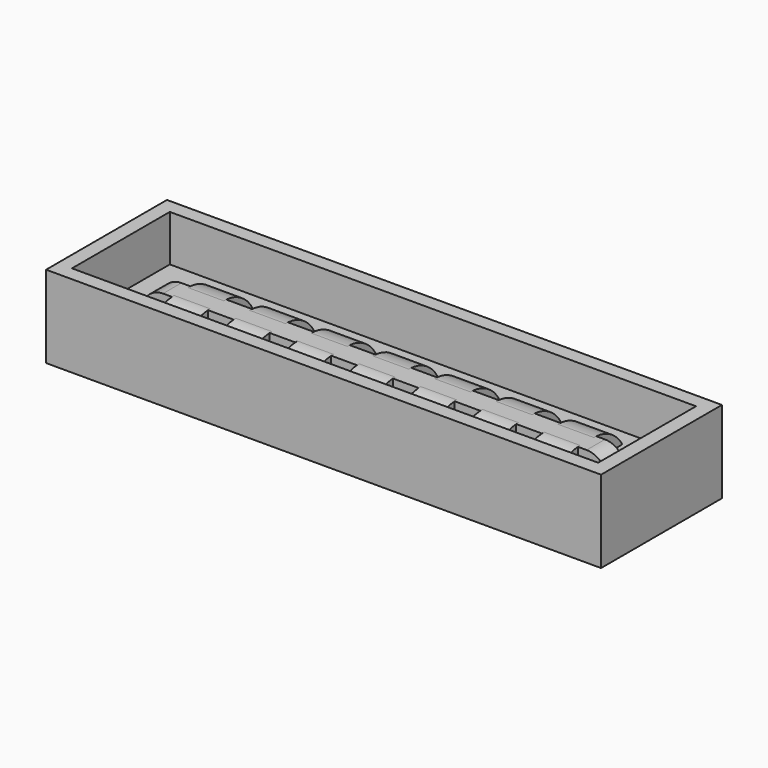
from build123d import *

# Parameters (mm, degrees)
F0_W         = 137.16
F0_H         = 37.338
F1_DEPTH     = 20.32
F2_W         = 130.048
F2_H         = 30.226
F3_DEPTH     = 11.43
F4_W         = 8.89
F4_H         = 21.844
F5_DEPTH     = 5.08
F6_T1_DEPTH  = 30.8870452561
F6_T3_DEPTH  = 52.8840905123
F6_T5_DEPTH  = 52.8840905123
F6_T7_DEPTH  = 52.8840905123
F6_T9_DEPTH  = 52.8840905123
F6_T11_DEPTH = 52.8840905123
F6_T13_DEPTH = 30.8870452561
F7_W         = 7.2538567698
F7_H         = 5.6681656279
F7_W_2       = 6.35
F8_DEPTH     = 5.08
F9_R         = 5.07999


# Not quite as in the source:
# - a fillet or chamfer that OpenCascade refuses, or shapes differently, is made with other operations: its cross-section is extruded or revolved along the edge and cut away or added
# - a fillet or chamfer is up to 0.001 mm smaller than in the source, because OpenCascade refuses the exact size
# - a feature names something its author has since deleted; it is built from what else it names


with BuildPart() as f1:
    # F0 (on Top) → F1 (new body)
    with BuildSketch(Plane.XY):
        Rectangle(F0_W, F0_H)
    extrude(amount=F1_DEPTH)

    # F2 (on face) → F3 (cut)
    with BuildSketch(Plane.XY.offset(20.32)):
        Rectangle(F2_W, F2_H)
    extrude(amount=-F3_DEPTH, mode=Mode.SUBTRACT)

    # F4 (on face) → F5 (join)
    with BuildSketch(Plane.XY.offset(8.89)):
        Rectangle(F4_W, F4_H)
        with Locations((15.24, 0)):
            Rectangle(F4_W, F4_H)
        with Locations((30.48, 0)):
            Rectangle(F4_W, F4_H)
        with Locations((45.72, 0)):
            Rectangle(F4_W, F4_H)
        with Locations((-15.24, 0)):
            Rectangle(F4_W, F4_H)
        with Locations((-30.48, 0)):
            Rectangle(F4_W, F4_H)
        with Locations((-45.72, 0)):
            Rectangle(F4_W, F4_H)
    extrude(amount=F5_DEPTH)

    # F6: fillet of radius 10.16 on 14 edges, made by hand

    # F6_s2 → F6_t1 (cut)
    with BuildSketch(Plane.YZ.offset(-50.165)):
        with BuildLine():
            ThreePointArc((-10.922, 8.89), (-7.2031818975, 12.6088181024), (-2.1231818975, 13.97))
            Line((-2.1231818975, 13.97), (-10.922, 13.97))
            Line((-10.922, 13.97), (-10.922, 8.89))
        make_face()
        with BuildLine():
            ThreePointArc((10.922, 8.89), (7.2031818975, 12.6088181024), (2.1231818975, 13.97))
            Line((2.1231818975, 13.97), (10.922, 13.97))
            Line((10.922, 13.97), (10.922, 8.89))
        make_face()
    extrude(amount=F6_T1_DEPTH, mode=Mode.SUBTRACT)

    # F6_s4 → F6_t3 (cut)
    with BuildSketch(Plane.YZ.offset(-56.9220452561)):
        with BuildLine():
            ThreePointArc((-10.922, 8.89), (-7.2031818975, 12.6088181024), (-2.1231818975, 13.97))
            Line((-2.1231818975, 13.97), (-10.922, 13.97))
            Line((-10.922, 13.97), (-10.922, 8.89))
        make_face()
        with BuildLine():
            ThreePointArc((10.922, 8.89), (7.2031818975, 12.6088181024), (2.1231818975, 13.97))
            Line((2.1231818975, 13.97), (10.922, 13.97))
            Line((10.922, 13.97), (10.922, 8.89))
        make_face()
    extrude(amount=F6_T3_DEPTH, mode=Mode.SUBTRACT)

    # F6_s6 → F6_t5 (cut)
    with BuildSketch(Plane.YZ.offset(-41.6820452561)):
        with BuildLine():
            ThreePointArc((-10.922, 8.89), (-7.2031818975, 12.6088181024), (-2.1231818975, 13.97))
            Line((-2.1231818975, 13.97), (-10.922, 13.97))
            Line((-10.922, 13.97), (-10.922, 8.89))
        make_face()
        with BuildLine():
            ThreePointArc((10.922, 8.89), (7.2031818975, 12.6088181024), (2.1231818975, 13.97))
            Line((2.1231818975, 13.97), (10.922, 13.97))
            Line((10.922, 13.97), (10.922, 8.89))
        make_face()
    extrude(amount=F6_T5_DEPTH, mode=Mode.SUBTRACT)

    # F6_s8 → F6_t7 (cut)
    with BuildSketch(Plane.YZ.offset(-26.4420452561)):
        with BuildLine():
            ThreePointArc((-10.922, 8.89), (-7.2031818975, 12.6088181024), (-2.1231818975, 13.97))
            Line((-2.1231818975, 13.97), (-10.922, 13.97))
            Line((-10.922, 13.97), (-10.922, 8.89))
        make_face()
        with BuildLine():
            ThreePointArc((10.922, 8.89), (7.2031818975, 12.6088181024), (2.1231818975, 13.97))
            Line((2.1231818975, 13.97), (10.922, 13.97))
            Line((10.922, 13.97), (10.922, 8.89))
        make_face()
    extrude(amount=F6_T7_DEPTH, mode=Mode.SUBTRACT)

    # F6_s10 → F6_t9 (cut)
    with BuildSketch(Plane.YZ.offset(-11.2020452561)):
        with BuildLine():
            ThreePointArc((-10.922, 8.89), (-7.2031818975, 12.6088181024), (-2.1231818975, 13.97))
            Line((-2.1231818975, 13.97), (-10.922, 13.97))
            Line((-10.922, 13.97), (-10.922, 8.89))
        make_face()
        with BuildLine():
            ThreePointArc((10.922, 8.89), (7.2031818975, 12.6088181024), (2.1231818975, 13.97))
            Line((2.1231818975, 13.97), (10.922, 13.97))
            Line((10.922, 13.97), (10.922, 8.89))
        make_face()
    extrude(amount=F6_T9_DEPTH, mode=Mode.SUBTRACT)

    # F6_s12 → F6_t11 (cut)
    with BuildSketch(Plane.YZ.offset(4.0379547439)):
        with BuildLine():
            ThreePointArc((-10.922, 8.89), (-7.2031818975, 12.6088181024), (-2.1231818975, 13.97))
            Line((-2.1231818975, 13.97), (-10.922, 13.97))
            Line((-10.922, 13.97), (-10.922, 8.89))
        make_face()
        with BuildLine():
            ThreePointArc((10.922, 8.89), (7.2031818975, 12.6088181024), (2.1231818975, 13.97))
            Line((2.1231818975, 13.97), (10.922, 13.97))
            Line((10.922, 13.97), (10.922, 8.89))
        make_face()
    extrude(amount=F6_T11_DEPTH, mode=Mode.SUBTRACT)

    # F6_s14 → F6_t13 (cut)
    with BuildSketch(Plane.YZ.offset(19.2779547439)):
        with BuildLine():
            ThreePointArc((-10.922, 8.89), (-7.2031818975, 12.6088181024), (-2.1231818975, 13.97))
            Line((-2.1231818975, 13.97), (-10.922, 13.97))
            Line((-10.922, 13.97), (-10.922, 8.89))
        make_face()
        with BuildLine():
            ThreePointArc((10.922, 8.89), (7.2031818975, 12.6088181024), (2.1231818975, 13.97))
            Line((2.1231818975, 13.97), (10.922, 13.97))
            Line((10.922, 13.97), (10.922, 8.89))
        make_face()
    extrude(amount=F6_T13_DEPTH, mode=Mode.SUBTRACT)

    # F7 (on face) → F8 (join)
    with BuildSketch(Plane.XY.offset(8.89)):
        with Locations((-53.7919283849, 0)):
            Rectangle(F7_W, F7_H)
        with Locations((-38.1, 0)):
            Rectangle(F7_W_2, F7_H)
        with Locations((-22.86, 0)):
            Rectangle(F7_W_2, F7_H)
        with Locations((-7.62, 0)):
            Rectangle(F7_W_2, F7_H)
        with Locations((7.62, 0)):
            Rectangle(F7_W_2, F7_H)
        with Locations((22.86, 0)):
            Rectangle(F7_W_2, F7_H)
        with Locations((38.1, 0)):
            Rectangle(F7_W_2, F7_H)
        with Locations((53.7919283849, 0)):
            Rectangle(F7_W, F7_H)
    extrude(amount=F8_DEPTH)

    # F9 (radius 5.08 in the source; OpenCascade refuses exactly that, so slightly less here)
    f9_edges = [f1.edges().sort_by_distance(p)[0] for p in [
        (-57.418857, 0, 13.97),
        (57.418857, 0, 13.97),
    ]]
    fillet(f9_edges, radius=F9_R)


solid = f1.part
